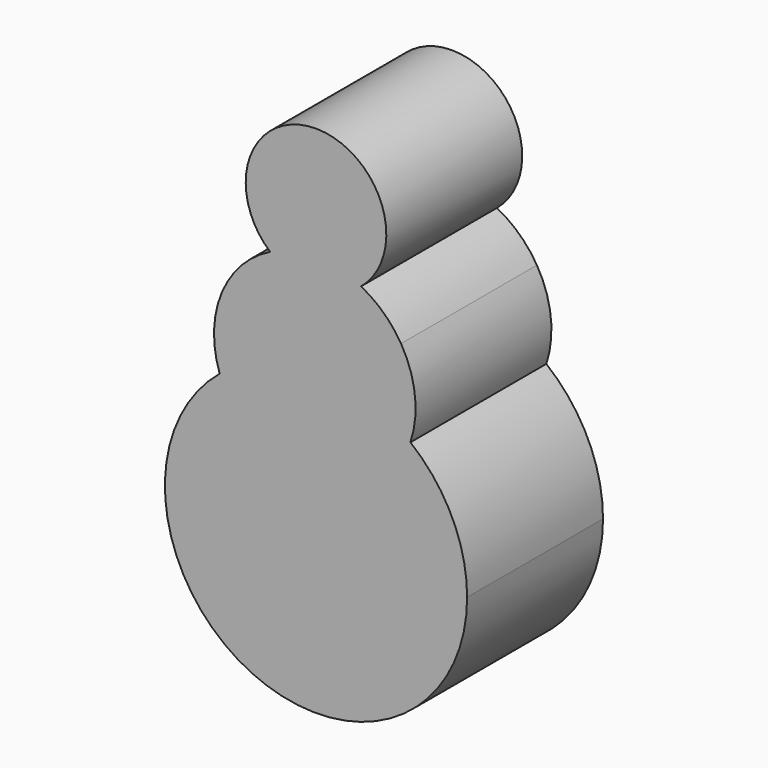
from build123d import *

# Parameters (mm, degrees)
F1_DEPTH = 25.4


with BuildPart() as f1:
    # F0 (on Front) → F1 (new body)
    with BuildSketch(Plane.XZ):
        with BuildLine():
            ThreePointArc((-14.4099858393, -36.15015585), (-9.6174010791, -74.0035828929), (22.5965727608, -53.5558275878))
            ThreePointArc((22.5965727608, -53.5558275878), (20.3675773267, -43.7697714683), (14.1203409545, -35.9143686951))
            ThreePointArc((14.1203409545, -35.9143686951), (-0.1867416275, -30.9600264713), (-14.4099858393, -36.15015585))
        make_face()
        with BuildLine():
            ThreePointArc((-14.4099858393, -36.15015585), (-0.1867416275, -30.9600264713), (14.1203409545, -35.9143686951))
            ThreePointArc((14.1203409545, -35.9143686951), (14.7921035223, -29.4911375194), (12.7136237721, -23.3764759904))
            ThreePointArc((12.7136237721, -23.3764759904), (10.1115297439, -20.1661301682), (6.7352958132, -17.7832205863))
            ThreePointArc((6.7352958132, -17.7832205863), (-0.0550758769, -16.1010168), (-6.8734396529, -17.6659042354))
            ThreePointArc((-6.8734396529, -17.6659042354), (-9.8053911529, -19.5704448334), (-12.2196112726, -22.0993093418))
            ThreePointArc((-12.2196112726, -22.0993093418), (-15.0762108242, -28.8501475286), (-14.4099858393, -36.15015585))
        make_face()
        with BuildLine():
            ThreePointArc((-6.8734396529, -17.6659042354), (-0.0550758769, -16.1010168), (6.7352958132, -17.7832205863))
            ThreePointArc((6.7352958132, -17.7832205863), (0.0906184951, 0.7995784888), (-6.8734396529, -17.6659042354))
        make_face()
    extrude(amount=F1_DEPTH)


solid = f1.part
